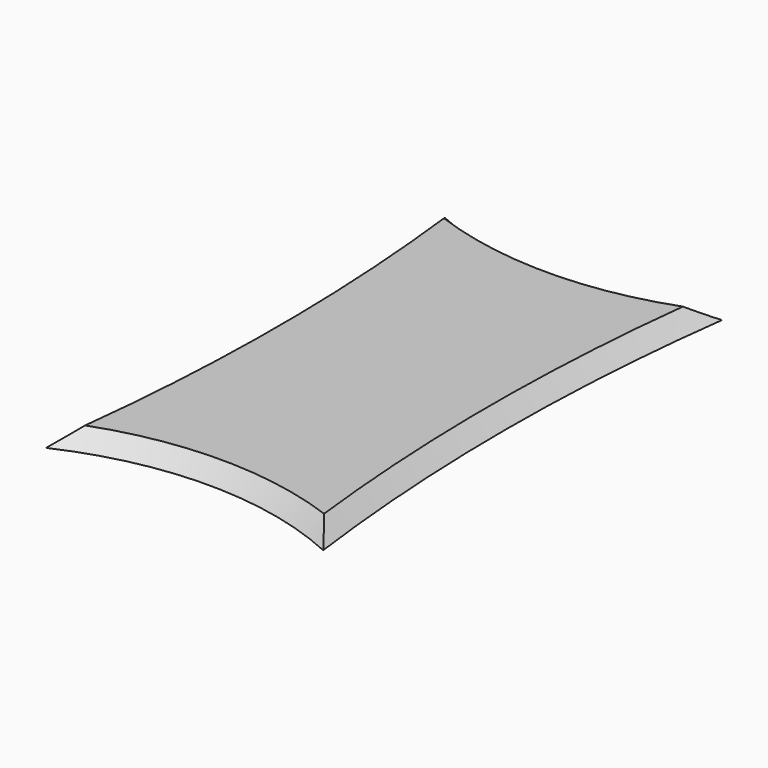
from build123d import *

# Parameters (mm, degrees)
F1_DEPTH    = 2.54
F2_T2_ANGLE = 21.6826985027
F2_T4_ANGLE = 89.4745768315
F2_T6_ANGLE = 21.6826985027
F2_T8_ANGLE = 89.4745768315


# Not quite as in the source:
# - a fillet or chamfer that OpenCascade refuses, or shapes differently, is made with other operations: its cross-section is extruded or revolved along the edge and cut away or added


with BuildPart() as f1:
    # F0 (on Top) → F1 (new body)
    with BuildSketch(Plane.XY):
        with BuildLine():
            ThreePointArc((-61.014207387, 8.6620835405), (-35.614207387, 15.4679930283), (-10.214207387, 8.6620835405))
            ThreePointArc((-10.214207387, 8.6620835405), (-13.4727715941, 53.1120835405), (-10.214207387, 97.5620835405))
            ThreePointArc((-10.214207387, 97.5620835405), (-35.614207387, 90.7561740528), (-61.014207387, 97.5620835405))
            ThreePointArc((-61.014207387, 97.5620835405), (-57.7556431798, 53.1120835405), (-61.014207387, 8.6620835405))
        make_face()
    extrude(amount=F1_DEPTH)

    # F2: chamfer of 5.08 on 4 edges, made by hand

    # F2_s1 → F2_t2 (revolve, cut)
    with BuildSketch(Plane(origin=(-22.6380198494, 118.2091118696, 0), x_dir=(0, 0, 1), z_dir=(-0.1880901634, 0.9821517655, 0))):
        Polygon((-2.54, -41.2948045664), (2.54, -36.2148045664), (2.54, -41.2948045664), align=None)
    revolve(axis=Axis((-362.5556431798, 53.1120835405, 2.54), (0, 0, -1)), revolution_arc=F2_T2_ANGLE, mode=Mode.SUBTRACT)

    # F2_s3 → F2_t4 (revolve, cut)
    with BuildSketch(Plane(origin=(-35.6356597066, -35.3103570189, 0), x_dir=(0, 0, 1), z_dir=(-0.7103415501, -0.7038571461, 0))):
        Polygon((-2.54, 50.7695217705), (2.54, 55.8495217705), (2.54, 50.7695217705), align=None)
    revolve(axis=Axis((-35.614207387, -35.3320069717, 2.54), (0, 0, -1)), revolution_arc=F2_T4_ANGLE, mode=Mode.SUBTRACT)

    # F2_s5 → F2_t6 (revolve, cut)
    with BuildSketch(Plane(origin=(0.4949892397, -2.5846888907, 0), x_dir=(0, 0, 1), z_dir=(0.1880901634, -0.9821517655, 0))):
        Polygon((-2.54, 8.6825878175), (2.54, 13.7625878175), (2.54, 8.6825878175), align=None)
    revolve(axis=Axis((291.3272284059, 53.1120835405, 2.54), (0, 0, -1)), revolution_arc=F2_T6_ANGLE, mode=Mode.SUBTRACT)

    # F2_s7 → F2_t8 (revolve, cut)
    with BuildSketch(Plane(origin=(52.8047119531, 52.3226803348, 0), x_dir=(0, 0, 1), z_dir=(0.7103415501, 0.7038571461, 0))):
        Polygon((-2.54, -74.8205464818), (2.54, -69.7405464818), (2.54, -74.8205464818), align=None)
    revolve(axis=Axis((-35.614207387, 141.5561740528, 2.54), (0, 0, -1)), revolution_arc=F2_T8_ANGLE, mode=Mode.SUBTRACT)


solid = f1.part
